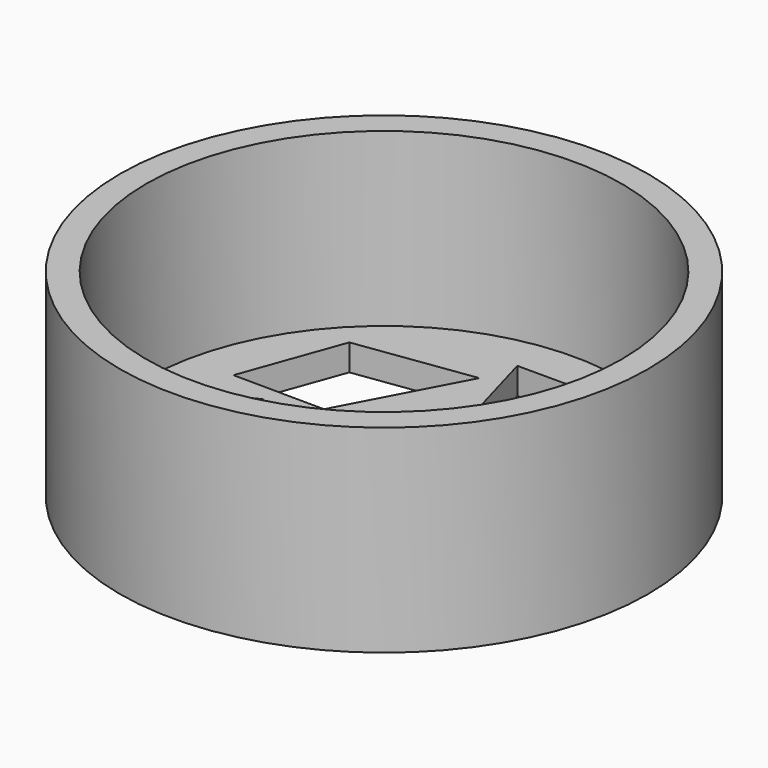
from build123d import *

# Parameters (mm, degrees)
F0_R      = 20
F1_DEPTH  = 15
F2_R      = 18
F3_DEPTH  = 13
F9_DEPTH  = 8.7
F11_DEPTH = 11
F13_DEPTH = 22.4
F14_DEPTH = 4.9


# Not quite as in the source:
# - the program builds the solid bodies; features that only make, move or delete a surface that nothing else refers to are left out


with BuildPart() as f1:
    # F0 (on Top) → F1 (new body)
    with BuildSketch(Plane.XY):
        Circle(F0_R)
    extrude(amount=F1_DEPTH)

    # F2 (on face) → F3 (cut)
    with BuildSketch(Plane.XY.offset(15)):
        Circle(F2_R)
    extrude(amount=-F3_DEPTH, mode=Mode.SUBTRACT)

    # F8 (on face) → F9 (cut)
    with BuildSketch(Plane(origin=(0, 0, 0), x_dir=(1, 0, 0), z_dir=(0, 0, -1))):
        Polygon((-11.5306517109, 11.1294062808), (-14.2554212362, 3.5755613353), (-7.3548774235, 3.5121154506), (-2.6781838387, 12.3627316207), align=None)
        Polygon((7.3548774235, 3.5121154506), (14.2554212362, 3.5755613353), (11.5306517109, 11.1294062808), (2.6781838387, 12.3627316207), align=None)
        Polygon((11.5306517109, -11.1294062808), (14.2554212362, -3.5755613353), (7.3548774235, -3.5121154506), (2.6781838387, -12.3627316207), align=None)
        Polygon((-14.2554212362, -3.5755613353), (-11.5306517109, -11.1294062808), (-2.6781838387, -12.3627316207), (-7.3548774235, -3.5121154506), align=None)
    extrude(amount=-F9_DEPTH, mode=Mode.SUBTRACT)

    # F10 (on face) → F11 (cut)
    with BuildSketch(Plane(origin=(0, 0, 0), x_dir=(1, 0, 0), z_dir=(0, 0, -1))):
        Polygon((15.5360468029, 0), (13.8570014387, 0.8311709389), (10.9741548076, 2.2582546808), (7.3600309273, 0), (10.9741548076, -2.2582546808), (13.8570014387, -0.8311709389), align=None)
        Polygon((-10.9741548076, -2.2582546808), (-7.3600309273, 0), (-10.9741548076, 2.2582546808), (-13.8570014387, 0.8311709389), (-15.5360468029, 0), (-13.8570014387, -0.8311709389), align=None)
    extrude(amount=-F11_DEPTH, mode=Mode.SUBTRACT)

    # F12 (on face) → F13 (cut)
    with BuildSketch(Plane.XY.offset(2)):
        Polygon((2.2074584849, 14.9893220514), (-1.9000733737, 14.9893220514), (0, 8.2467701286), align=None)
        Polygon((-1.9000733737, -14.9893220514), (2.2074584849, -14.9893220514), (0, -8.2467701286), align=None)
    extrude(amount=F13_DEPTH, mode=Mode.SUBTRACT)

    # F12 (on face) → F14 (cut)
    with BuildSketch(Plane.XY.offset(2)):
        Polygon((2.2074584849, 14.9893220514), (-1.9000733737, 14.9893220514), (0, 8.2467701286), align=None)
        Polygon((-1.9000733737, -14.9893220514), (2.2074584849, -14.9893220514), (0, -8.2467701286), align=None)
    extrude(amount=-F14_DEPTH, mode=Mode.SUBTRACT)


solid = f1.part
